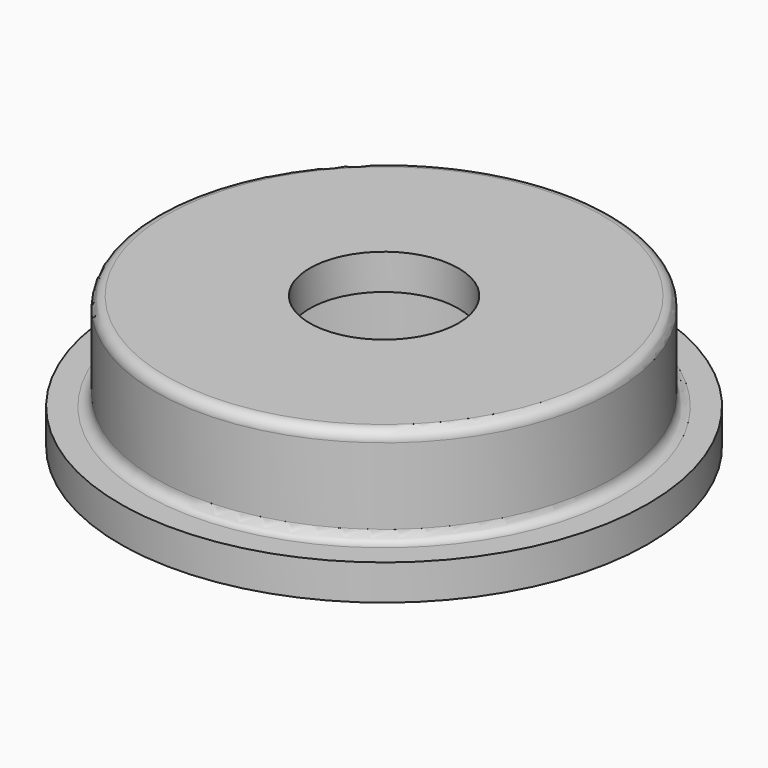
from build123d import *

# Parameters (mm, degrees)
F2_R = 0.762


with BuildPart() as f1:
    # F0 (on Front) → F1 (revolve)
    with BuildSketch(Plane.XZ):
        Polygon((-39.4238941371, 11.021196073), (-39.4238941371, 8.481196073), (-33.6445995694, 8.481196073), (-33.6445995694, 1.496196073), (-25.8340995694, 1.496196073), (-25.8340995694, 4.036196073), (-28.3740995694, 4.036196073), (-28.3740995694, 11.021196073), align=None)
    revolve(axis=Axis((-44.7570995694, 0, 2.9726716104), (0, 0, -1)))

    # F2
    f2_edges = [f1.edges().sort_by_distance(p)[0] for p in [
        (-61.1401, 0, 11.021196),
        (-61.1401, 0, 4.036196),
        (-28.3741, 0, 7.528696),
    ]]
    fillet(f2_edges, radius=F2_R)


solid = f1.part
